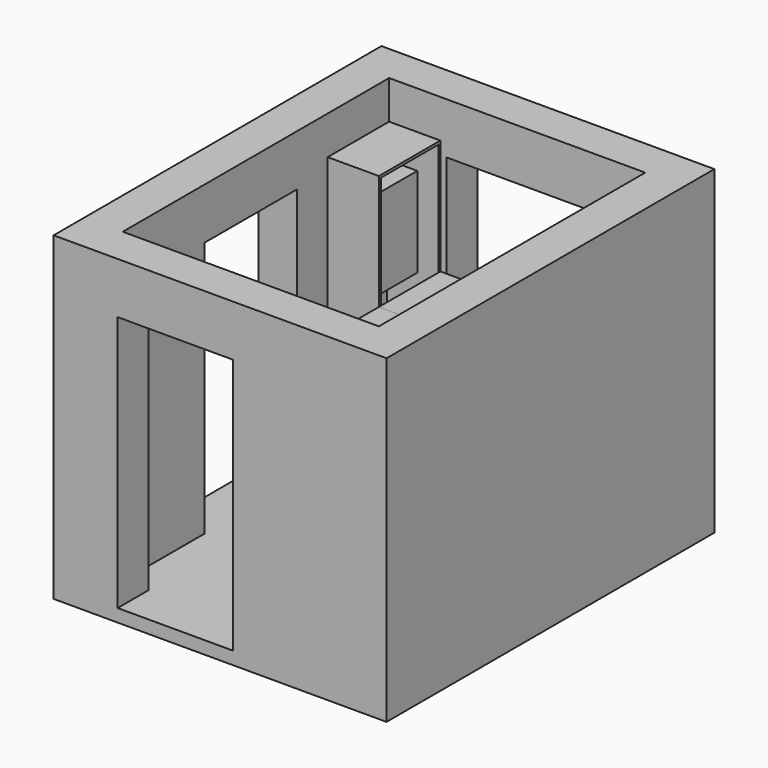
from build123d import *

# Parameters (mm, degrees)
F1_DEPTH  = 2400
F2_DEPTH  = 100
F3_W      = 600
F3_H      = 600
F4_DEPTH  = 850
F5_DEPTH  = 850
F6_DEPTH  = 2000
F7_DEPTH  = 2000
F3_W_2    = 10
F3_H_2    = 200
F8_DEPTH  = 2000
F9_W      = 600
F9_H      = 1000
F10_DEPTH = 300
F9_W_2    = 900
F9_H_2    = 400
F11_DEPTH = 300
F12_W     = 900
F12_H     = 400
F13_DEPTH = 300
F14_W     = 900
F14_H     = 2000
F15_DEPTH = 300
F16_W     = 1000
F16_H     = 720
F17_DEPTH = 300
F18_W     = 390
F18_H     = 700
F19_DEPTH = 300
F20_W     = 600
F20_H     = 2100
F20_W_2   = 560
F20_H_2   = 2060
F21_DEPTH = 400
F22_W     = 600
F22_H     = 900
F23_DEPTH = 660
F24_W     = 1800
F24_H     = 35
F25_DEPTH = 660


# Not quite as in the source:
# - a feature names something its author has since deleted; it is built from what else it names


with BuildPart() as f1:
    # F0 (on Top) → F1 (new body)
    with BuildSketch(Plane.XY):
        Polygon((1300, 1600), (350, 1600), (350, 1300), (1000, 1300), (1000, -1300), (100, -1300), (100, -1600), (1300, -1600), align=None)
    extrude(amount=F1_DEPTH)



with BuildPart() as f1b:
    # F0 (on Top) → F1, piece 2 (new body)
    with BuildSketch(Plane.XY):
        Polygon((-1000, -1300), (-1000, 1300), (-550, 1300), (-550, 1600), (-1300, 1600), (-1300, -1600), (-800, -1600), (-800, -1300), align=None)
    extrude(amount=F1_DEPTH)


with BuildPart() as f1_1:
    add(f1.part)

    add(f1b.part)  # F2 merges F1b
    # F0 (on Top) → F2 (join)
    with BuildSketch(Plane.XY):
        Polygon((-550, 1300), (-1000, 1300), (-1000, -1300), (-800, -1300), (-800, -1600), (100, -1600), (100, -1300), (1000, -1300), (1000, 1300), (350, 1300), (350, 1600), (-550, 1600), align=None)
        Polygon((-1000, -1300), (-1000, 1300), (-550, 1300), (-550, 1600), (-1300, 1600), (-1300, -1600), (-800, -1600), (-800, -1300), align=None)
        Polygon((1300, 1600), (350, 1600), (350, 1300), (1000, 1300), (1000, -1300), (100, -1300), (100, -1600), (1300, -1600), align=None)
    extrude(amount=-F2_DEPTH)

    # F9 (on face) → F10 (cut, through all)
    with BuildSketch(Plane(origin=(0, 1600, 0), x_dir=(-1, 0, 0), z_dir=(0, 1, 0))):
        with Locations((-650, 1500)):
            Rectangle(F9_W, F9_H)
    extrude(amount=-F10_DEPTH, mode=Mode.SUBTRACT)

    # F9 (on face) → F11 (join, through all)
    with BuildSketch(Plane(origin=(0, 1600, 0), x_dir=(-1, 0, 0), z_dir=(0, 1, 0))):
        with Locations((100, 2200)):
            Rectangle(F9_W_2, F9_H_2)
    extrude(amount=-F11_DEPTH)

    # F12 (on face) → F13 (join, through all)
    with BuildSketch(Plane.XZ.offset(1600)):
        with Locations((-350, 2200)):
            Rectangle(F12_W, F12_H)
    extrude(amount=-F13_DEPTH)

    # F14 (on face) → F15 (cut, through all)
    with BuildSketch(Plane(origin=(-1300, 0, 0), x_dir=(0, -1, 0), z_dir=(-1, 0, 0))):
        with Locations((50, 1000)):
            Rectangle(F14_W, F14_H)
    extrude(amount=-F15_DEPTH, mode=Mode.SUBTRACT)


with BuildPart() as f4:
    # F3 (on face) → F4 (new body)
    with BuildSketch(Plane.XY):
        with Locations((660, 1000)):
            Rectangle(F3_W, F3_H)
    extrude(amount=F4_DEPTH)


with BuildPart() as f5:
    # F3 (on face) → F5 (new body)
    with BuildSketch(Plane.XY):
        with Locations((660, 400)):
            Rectangle(F3_W, F3_H)
    extrude(amount=F5_DEPTH)


with BuildPart() as f6:
    # F3 (on face) → F6 (new body)
    with BuildSketch(Plane.XY):
        with Locations((660, -200)):
            Rectangle(F3_W, F3_H)
    extrude(amount=F6_DEPTH)


with BuildPart() as f7:
    # F3 (on face) → F7 (new body)
    with BuildSketch(Plane.XY):
        Polygon((960, -1100), (960, -500), (360, -500), (360, -1100), (370, -1100), align=None)
    extrude(amount=F7_DEPTH)


with BuildPart() as f8:
    # F3 (on face) → F8 (new body)
    with BuildSketch(Plane.XY):
        with Locations((365, -1200)):
            Rectangle(F3_W_2, F3_H_2)
    extrude(amount=F8_DEPTH)


with BuildPart() as f17:
    # F16 (on face) → F17 (new body)
    with BuildSketch(Plane(origin=(1000, 0, 0), x_dir=(0, -1, 0), z_dir=(-1, 0, 0))):
        with Locations((0, 1640)):
            Rectangle(F16_W, F16_H)
    extrude(amount=F17_DEPTH)


with BuildPart() as f19:
    # F18 (on face) → F19 (new body)
    with BuildSketch(Plane.YZ.offset(-1000)):
        with Locations((1005, 1550)):
            Rectangle(F18_W, F18_H)
    extrude(amount=F19_DEPTH)


with BuildPart() as f21:
    # F20 (on face) → F21 (new body)
    with BuildSketch(Plane.YZ.offset(-1000)):
        with Locations((1000, 1050)):
            Rectangle(F20_W, F20_H)
        with Locations((1000, 1050)):
            Rectangle(F20_W_2, F20_H_2, mode=Mode.SUBTRACT)
    extrude(amount=F21_DEPTH)


with BuildPart() as f23:
    # F22 (on face) → F23 (new body)
    with BuildSketch(Plane(origin=(1000, 0, 0), x_dir=(0, -1, 0), z_dir=(-1, 0, 0))):
        with Locations((200, 450)):
            Rectangle(F22_W, F22_H)
    extrude(amount=F23_DEPTH)


with BuildPart() as f25:
    # F24 (on face) → F25 (new body, through all)
    with BuildSketch(Plane(origin=(1000, 0, 0), x_dir=(0, -1, 0), z_dir=(-1, 0, 0))):
        with Locations((-400, 917.5)):
            Rectangle(F24_W, F24_H)
    extrude(amount=F25_DEPTH)


solid = Compound([f1_1.part, f4.part, f5.part, f6.part, f7.part, f8.part, f17.part, f19.part, f21.part, f23.part, f25.part])
